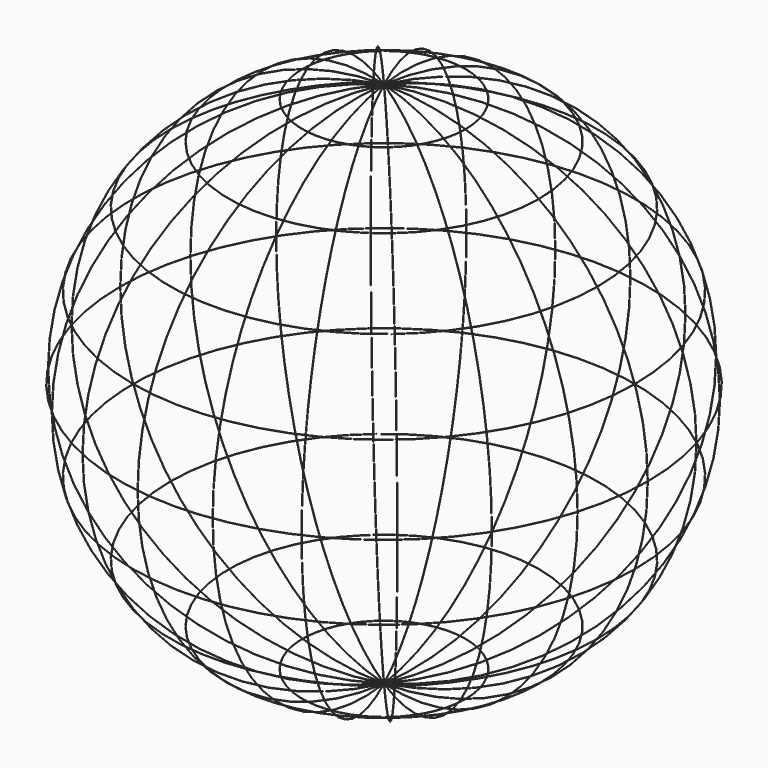
from build123d import *

# Parameters (mm, degrees)
F0_R     = 0.05
F2_R     = 0.05
F4_COUNT = 22


with BuildPart() as f1:
    # F0 (on Front) → F1 (revolve)
    with BuildSketch(Plane.XZ):
        with Locations((60.5374964603, 43.9830657174)):
            Circle(F0_R)
    revolve(axis=Axis((0, 0, 37.4142304063), (0, 0, 1)))


with BuildPart() as f1b:
    # F0 (on Front) → F1, piece 2 (revolve)
    with BuildSketch(Plane.XZ):
        with Locations((23.123266054, 71.1660952601)):
            Circle(F0_R)
    revolve(axis=Axis((0, 0, 37.4142304063), (0, 0, 1)))


with BuildPart() as f1c:
    # F0 (on Front) → F1, piece 3 (revolve)
    with BuildSketch(Plane.XZ):
        with Locations((60.5374964603, -43.9830657174)):
            Circle(F0_R)
    revolve(axis=Axis((0, 0, 37.4142304063), (0, 0, 1)))


with BuildPart() as f1d:
    # F0 (on Front) → F1, piece 4 (revolve)
    with BuildSketch(Plane.XZ):
        with Locations((43.9830657174, 60.5374964603)):
            Circle(F0_R)
    revolve(axis=Axis((0, 0, 37.4142304063), (0, 0, 1)))


with BuildPart() as f1e:
    # F0 (on Front) → F1, piece 5 (revolve)
    with BuildSketch(Plane.XZ):
        with Locations((23.123266054, -71.1660952601)):
            Circle(F0_R)
    revolve(axis=Axis((0, 0, 37.4142304063), (0, 0, 1)))


with BuildPart() as f1f:
    # F0 (on Front) → F1, piece 6 (revolve)
    with BuildSketch(Plane.XZ):
        with Locations((71.1660952601, 23.123266054)):
            Circle(F0_R)
    revolve(axis=Axis((0, 0, 37.4142304063), (0, 0, 1)))


with BuildPart() as f1g:
    # F0 (on Front) → F1, piece 7 (revolve)
    with BuildSketch(Plane.XZ):
        with Locations((71.1660952601, -23.123266054)):
            Circle(F0_R)
    revolve(axis=Axis((0, 0, 37.4142304063), (0, 0, 1)))


with BuildPart() as f1h:
    # F0 (on Front) → F1, piece 8 (revolve)
    with BuildSketch(Plane.XZ):
        with Locations((43.9830657174, -60.5374964603)):
            Circle(F0_R)
    revolve(axis=Axis((0, 0, 37.4142304063), (0, 0, 1)))


with BuildPart() as f1i:
    # F0 (on Front) → F1, piece 9 (revolve)
    with BuildSketch(Plane.XZ):
        with Locations((74.8284608126, 0)):
            Circle(F0_R)
    revolve(axis=Axis((0, 0, 37.4142304063), (0, 0, 1)))


with BuildPart() as f3:
    # F3: sweep along a path in F0
    with BuildLine(Plane.XZ) as f3_path:
        ThreePointArc((0, 74.8284608126), (-74.8284566364, -0.025), (0.0499999972, -74.8284441077))
    # F2 (on Right) → F3 (sweep)
    with BuildSketch(Plane.YZ):
        with Locations((0, 74.8284757137)):
            Circle(F2_R)
    sweep(path=f3_path.line)


with BuildPart() as f4_1:
    # F4: instance of F3
    add(f3.part.rotate(Axis((0, 0, 37.4142304063), (0, 0, 1)), 1 * 360 / F4_COUNT))


with BuildPart() as f4_2:
    # F4: instance of F3
    add(f3.part.rotate(Axis((0, 0, 37.4142304063), (0, 0, 1)), 2 * 360 / F4_COUNT))


with BuildPart() as f4_3:
    # F4: instance of F3
    add(f3.part.rotate(Axis((0, 0, 37.4142304063), (0, 0, 1)), 3 * 360 / F4_COUNT))


with BuildPart() as f4_4:
    # F4: instance of F3
    add(f3.part.rotate(Axis((0, 0, 37.4142304063), (0, 0, 1)), 4 * 360 / F4_COUNT))


with BuildPart() as f4_5:
    # F4: instance of F3
    add(f3.part.rotate(Axis((0, 0, 37.4142304063), (0, 0, 1)), 5 * 360 / F4_COUNT))


with BuildPart() as f4_6:
    # F4: instance of F3
    add(f3.part.rotate(Axis((0, 0, 37.4142304063), (0, 0, 1)), 6 * 360 / F4_COUNT))


with BuildPart() as f4_7:
    # F4: instance of F3
    add(f3.part.rotate(Axis((0, 0, 37.4142304063), (0, 0, 1)), 7 * 360 / F4_COUNT))


with BuildPart() as f4_8:
    # F4: instance of F3
    add(f3.part.rotate(Axis((0, 0, 37.4142304063), (0, 0, 1)), 8 * 360 / F4_COUNT))


with BuildPart() as f4_9:
    # F4: instance of F3
    add(f3.part.rotate(Axis((0, 0, 37.4142304063), (0, 0, 1)), 9 * 360 / F4_COUNT))


with BuildPart() as f4_10:
    # F4: instance of F3
    add(f3.part.rotate(Axis((0, 0, 37.4142304063), (0, 0, 1)), 10 * 360 / F4_COUNT))


with BuildPart() as f4_11:
    # F4: instance of F3
    add(f3.part.rotate(Axis((0, 0, 37.4142304063), (0, 0, 1)), 11 * 360 / F4_COUNT))


with BuildPart() as f4_12:
    # F4: instance of F3
    add(f3.part.rotate(Axis((0, 0, 37.4142304063), (0, 0, 1)), 12 * 360 / F4_COUNT))


with BuildPart() as f4_13:
    # F4: instance of F3
    add(f3.part.rotate(Axis((0, 0, 37.4142304063), (0, 0, 1)), 13 * 360 / F4_COUNT))


with BuildPart() as f4_14:
    # F4: instance of F3
    add(f3.part.rotate(Axis((0, 0, 37.4142304063), (0, 0, 1)), 14 * 360 / F4_COUNT))


with BuildPart() as f4_15:
    # F4: instance of F3
    add(f3.part.rotate(Axis((0, 0, 37.4142304063), (0, 0, 1)), 15 * 360 / F4_COUNT))


with BuildPart() as f4_16:
    # F4: instance of F3
    add(f3.part.rotate(Axis((0, 0, 37.4142304063), (0, 0, 1)), 16 * 360 / F4_COUNT))


with BuildPart() as f4_17:
    # F4: instance of F3
    add(f3.part.rotate(Axis((0, 0, 37.4142304063), (0, 0, 1)), 17 * 360 / F4_COUNT))


with BuildPart() as f4_18:
    # F4: instance of F3
    add(f3.part.rotate(Axis((0, 0, 37.4142304063), (0, 0, 1)), 18 * 360 / F4_COUNT))


with BuildPart() as f4_19:
    # F4: instance of F3
    add(f3.part.rotate(Axis((0, 0, 37.4142304063), (0, 0, 1)), 19 * 360 / F4_COUNT))


with BuildPart() as f4_20:
    # F4: instance of F3
    add(f3.part.rotate(Axis((0, 0, 37.4142304063), (0, 0, 1)), 20 * 360 / F4_COUNT))


with BuildPart() as f4_21:
    # F4: instance of F3
    add(f3.part.rotate(Axis((0, 0, 37.4142304063), (0, 0, 1)), 21 * 360 / F4_COUNT))


solid = Compound([f1.part, f1b.part, f1c.part, f1d.part, f1e.part, f1f.part, f1g.part, f1h.part, f1i.part, f3.part, f4_1.part, f4_2.part, f4_3.part, f4_4.part, f4_5.part, f4_6.part, f4_7.part, f4_8.part, f4_9.part, f4_10.part, f4_11.part, f4_12.part, f4_13.part, f4_14.part, f4_15.part, f4_16.part, f4_17.part, f4_18.part, f4_19.part, f4_20.part, f4_21.part])
